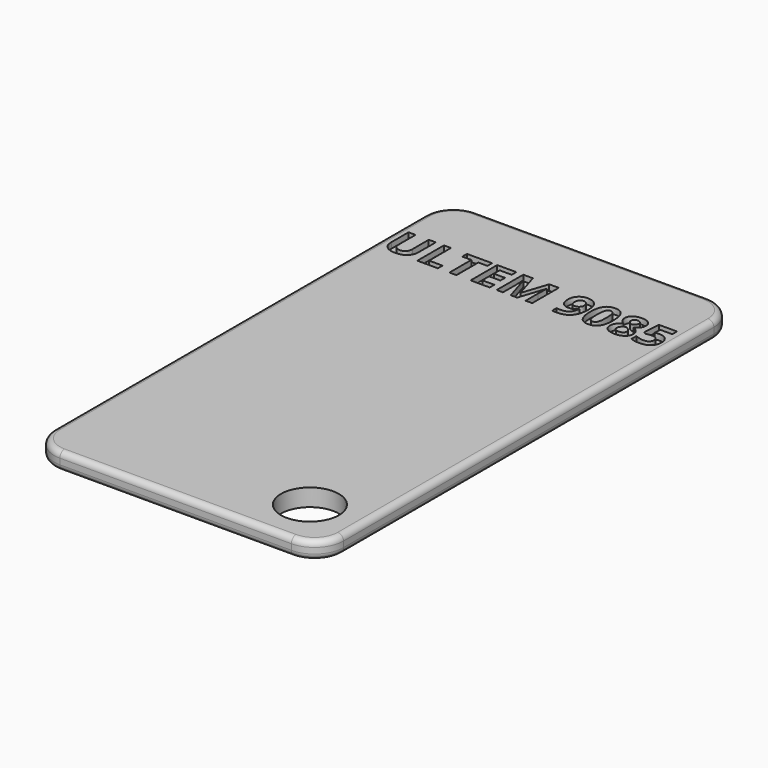
from build123d import *

# Parameters (mm, degrees)
F0_W         = 90
F0_H         = 50
F1_DEPTH     = 3
F2_R         = 1
F3_T1_DEPTH  = 3
F3_T4_ANGLE  = 90
F3_T6_ANGLE  = 90
F3_T8_ANGLE  = 90
F3_T10_ANGLE = 90
F3_T12_ANGLE = 90
F3_T14_ANGLE = 90
F3_T16_ANGLE = 90
F3_T18_ANGLE = 90
F5_ANGLE     = 90
F6_TEXT_SIZE = 8.0458866976
F7_DEPTH     = 1
F8_R         = 5
F9_DEPTH     = 3


# Not quite as in the source:
# - a fillet or chamfer that OpenCascade refuses, or shapes differently, is made with other operations: its cross-section is extruded or revolved along the edge and cut away or added
# - Text() gives the source's letters only with a copy of the font that has no kerning and outlines rounded to 1/6400 em; it was checked with that copy


with BuildPart() as f1:
    # F0 (on Top) → F1 (new body)
    with BuildSketch(Plane.XY):
        Rectangle(F0_W, F0_H)
    extrude(amount=F1_DEPTH)

    # F2
    f2_edges = [f1.edges().sort_by_distance(p)[0] for p in [
        (0, 25, 3),
        (-45, 0, 3),
        (0, -25, 3),
        (45, 0, 3),
        (0, 25, 0),
        (-45, 0, 0),
        (0, -25, 0),
        (45, 0, 0),
    ]]
    fillet(f2_edges, radius=F2_R)

    # F3: fillet of radius 5 on 4 edges, made by hand

    # F3_s2 → F3_t1 (cut)
    with BuildSketch(Plane.XY):
        with BuildLine():
            ThreePointArc((45, -20), (43.5355339059, -23.5355339059), (40, -25))
            Line((40, -25), (45, -25))
            Line((45, -25), (45, -20))
        make_face()
        with BuildLine():
            ThreePointArc((40, 25), (43.5355339059, 23.5355339059), (45, 20))
            Line((45, 20), (45, 25))
            Line((45, 25), (40, 25))
        make_face()
        with BuildLine():
            ThreePointArc((-40, 25), (-43.5355339059, 23.5355339059), (-45, 20))
            Line((-45, 20), (-45, 25))
            Line((-45, 25), (-40, 25))
        make_face()
        with BuildLine():
            ThreePointArc((-45, -20), (-43.5355339059, -23.5355339059), (-40, -25))
            Line((-40, -25), (-45, -25))
            Line((-45, -25), (-45, -20))
        make_face()
    extrude(amount=F3_T1_DEPTH, mode=Mode.SUBTRACT)

    # F3_s3 → F3_t4 (revolve, cut)
    with BuildSketch(Plane.YZ.offset(-40)):
        with BuildLine():
            ThreePointArc((-24, 0), (-24.7071067812, 0.2928932188), (-25, 1))
            Line((-25, 1), (-25, 0))
            Line((-25, 0), (-24, 0))
        make_face()
    revolve(axis=Axis((-40, -20, 0), (0, 0, -1)), revolution_arc=F3_T4_ANGLE, mode=Mode.SUBTRACT)

    # F3_s5 → F3_t6 (revolve, cut)
    with BuildSketch(Plane.XZ.offset(20)):
        with BuildLine():
            ThreePointArc((-44, 3), (-44.7071067812, 2.7071067812), (-45, 2))
            Line((-45, 2), (-45, 3))
            Line((-45, 3), (-44, 3))
        make_face()
    revolve(axis=Axis((-40, -20, 3), (0, 0, 1)), revolution_arc=F3_T6_ANGLE, mode=Mode.SUBTRACT)

    # F3_s7 → F3_t8 (revolve, cut)
    with BuildSketch(Plane.XZ.offset(-20)):
        with BuildLine():
            ThreePointArc((-44, 0), (-44.7071067812, 0.2928932188), (-45, 1))
            Line((-45, 1), (-45, 0))
            Line((-45, 0), (-44, 0))
        make_face()
    revolve(axis=Axis((-40, 20, 0), (0, 0, -1)), revolution_arc=F3_T8_ANGLE, mode=Mode.SUBTRACT)

    # F3_s9 → F3_t10 (revolve, cut)
    with BuildSketch(Plane.YZ.offset(-40)):
        with BuildLine():
            ThreePointArc((24, 3), (24.7071067812, 2.7071067812), (25, 2))
            Line((25, 2), (25, 3))
            Line((25, 3), (24, 3))
        make_face()
    revolve(axis=Axis((-40, 20, 3), (0, 0, 1)), revolution_arc=F3_T10_ANGLE, mode=Mode.SUBTRACT)

    # F3_s11 → F3_t12 (revolve, cut)
    with BuildSketch(Plane.YZ.offset(40)):
        with BuildLine():
            ThreePointArc((24, 0), (24.7071067812, 0.2928932188), (25, 1))
            Line((25, 1), (25, 0))
            Line((25, 0), (24, 0))
        make_face()
    revolve(axis=Axis((40, 20, 0), (0, 0, -1)), revolution_arc=F3_T12_ANGLE, mode=Mode.SUBTRACT)

    # F3_s13 → F3_t14 (revolve, cut)
    with BuildSketch(Plane.XZ.offset(-20)):
        with BuildLine():
            ThreePointArc((44, 3), (44.7071067812, 2.7071067812), (45, 2))
            Line((45, 2), (45, 3))
            Line((45, 3), (44, 3))
        make_face()
    revolve(axis=Axis((40, 20, 3), (0, 0, 1)), revolution_arc=F3_T14_ANGLE, mode=Mode.SUBTRACT)

    # F3_s15 → F3_t16 (revolve, cut)
    with BuildSketch(Plane.XZ.offset(20)):
        with BuildLine():
            ThreePointArc((44, 0), (44.7071067812, 0.2928932188), (45, 1))
            Line((45, 1), (45, 0))
            Line((45, 0), (44, 0))
        make_face()
    revolve(axis=Axis((40, -20, 0), (0, 0, -1)), revolution_arc=F3_T16_ANGLE, mode=Mode.SUBTRACT)

    # F3_s17 → F3_t18 (revolve, cut)
    with BuildSketch(Plane.YZ.offset(40)):
        with BuildLine():
            ThreePointArc((-24, 3), (-24.7071067812, 2.7071067812), (-25, 2))
            Line((-25, 2), (-25, 3))
            Line((-25, 3), (-24, 3))
        make_face()
    revolve(axis=Axis((40, -20, 3), (0, 0, 1)), revolution_arc=F3_T18_ANGLE, mode=Mode.SUBTRACT)


with BuildPart() as f1_1:
    # F5: moved
    add(f1.part.rotate(Axis((0, 0, 16.4477843791), (0, 0, 1)), F5_ANGLE))

    # F6 (on face) → F7 (cut)
    with BuildSketch(Plane.XY.offset(3)):
        with Locations((-24, 28.6923076827)):
            Text('ULTEM 9085', F6_TEXT_SIZE, font='Open Sans', font_style=FontStyle.BOLD, text_align=(TextAlign.LEFT, TextAlign.BOTTOM))
    extrude(amount=-F7_DEPTH, mode=Mode.SUBTRACT)

    # F8 (on face) → F9 (cut)
    with BuildSketch(Plane.XY.offset(3)):
        with Locations((16, -36)):
            Circle(F8_R)
    extrude(amount=-F9_DEPTH, mode=Mode.SUBTRACT)


solid = f1_1.part
